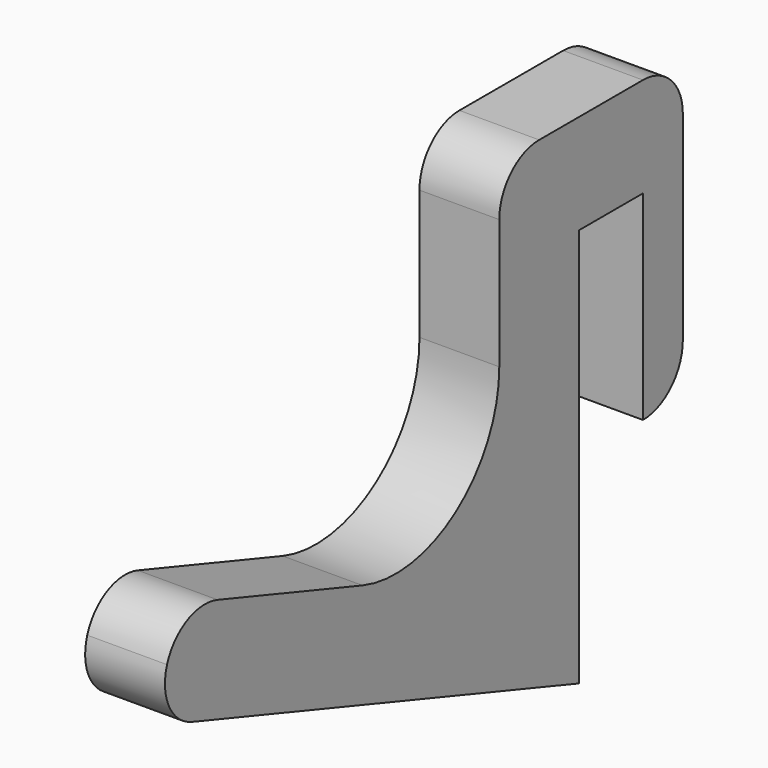
from build123d import *

# Parameters (mm, degrees)
F1_DEPTH = 8
F2_R     = 4.99999
F3_R     = 13
F4_R     = 4.99999


# Not quite as in the source:
# - a fillet or chamfer is up to 0.001 mm smaller than in the source, because OpenCascade refuses the exact size


with BuildPart() as f1:
    # F0 (on Right) → F1 (new body)
    with BuildSketch(Plane.YZ):
        Polygon((11.3393977799, 240.6016960415), (-11.6606022201, 240.6016960415), (-11.6606022201, 204.5172253872), (-51.7021150763, 217.9898196767), (-54.8910993051, 208.5119306929), (-1.6606022201, 190.6016960415), (-1.6606022201, 230.6016960415), (6.3393977799, 230.6016960415), (6.3393977799, 210.6016960415), (11.3393977799, 210.6016960415), align=None)
    extrude(amount=-F1_DEPTH)

    # F2 (radius 5 in the source; OpenCascade refuses exactly that, so slightly less here)
    f2_edges = [f1.edges().sort_by_distance(p)[0] for p in [
        (-4, -51.702115, 217.98982),
        (-4, -54.891099, 208.511931),
    ]]
    fillet(f2_edges, radius=F2_R)

    # F3
    f3_edges = [f1.edges().sort_by_distance(p)[0] for p in [
        (-4, -11.660602, 204.517225),
    ]]
    fillet(f3_edges, radius=F3_R)

    # F4 (radius 5 in the source; OpenCascade refuses exactly that, so slightly less here)
    f4_edges = [f1.edges().sort_by_distance(p)[0] for p in [
        (-4, -11.660602, 240.601696),
        (-4, 11.339398, 240.601696),
        (-4, 11.339398, 210.601696),
    ]]
    fillet(f4_edges, radius=F4_R)


solid = f1.part
